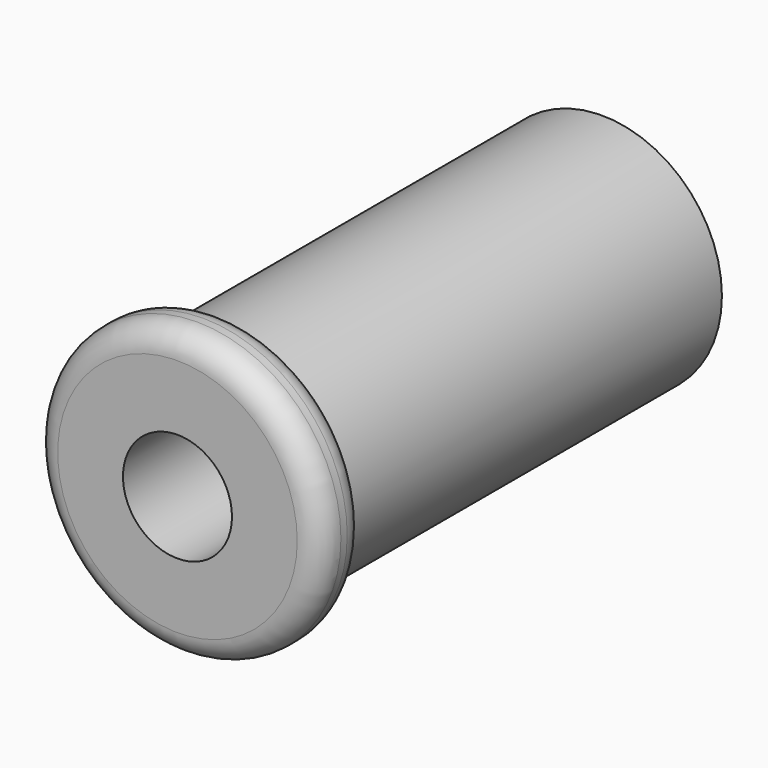
from build123d import *

# Parameters (mm, degrees)
F0_R        = 2.0088927205
F0_R_2      = 0.9130728347
F1_DEPTH    = 8.89
F0_R_3      = 2.413
F2_DEPTH    = 0.94454
F3_S5_R     = 2.0088927205
F3_T6_DEPTH = 5


# Not quite as in the source:
# - a fillet or chamfer that OpenCascade refuses, or shapes differently, is made with other operations: its cross-section is extruded or revolved along the edge and cut away or added


with BuildPart() as f1:
    # F0 (on Front) → F1 (new body)
    with BuildSketch(Plane.XZ):
        Circle(F0_R)
        Circle(F0_R_2, mode=Mode.SUBTRACT)
    extrude(amount=-F1_DEPTH)

    # F0 (on Front) → F2 (join)
    with BuildSketch(Plane.XZ):
        Circle(F0_R_3)
        Circle(F0_R, mode=Mode.SUBTRACT)
    extrude(amount=-F2_DEPTH)

    # F3: fillet of radius 0.4064 on 2 edges, made by hand


with BuildPart() as f3_tool2:
    # F3_s3 → F3_t4 (revolve)
    with BuildSketch(Plane.XY):
        with BuildLine():
            ThreePointArc((2.0066, 0.94454), (2.2939681959, 0.8255081959), (2.413, 0.53814))
            Line((2.413, 0.53814), (2.413, 0.94454))
            Line((2.413, 0.94454), (2.0066, 0.94454))
        make_face()
    revolve(axis=Axis((0, 0.94454, 0), (0, -1, 0)))

    # F3_s5 → F3_t6 (cut, symmetric)
    with BuildSketch(Plane.XZ.offset(-0.6)):
        Circle(F3_S5_R)
    extrude(amount=F3_T6_DEPTH, both=True, mode=Mode.SUBTRACT)


with BuildPart() as f1_1:
    add(f1.part)

    # F3_t1: cut F3_tool2
    add(f3_tool2.part, mode=Mode.SUBTRACT)

    # F3_s7 → F3_t8 (revolve, cut)
    with BuildSketch(Plane.XY):
        with BuildLine():
            ThreePointArc((2.413, 0.4064), (2.2939681959, 0.1190318041), (2.0066, 0))
            Line((2.0066, 0), (2.413, 0))
            Line((2.413, 0), (2.413, 0.4064))
        make_face()
    revolve(axis=Axis((0, 0, 0), (0, -1, 0)), mode=Mode.SUBTRACT)


solid = f1_1.part
